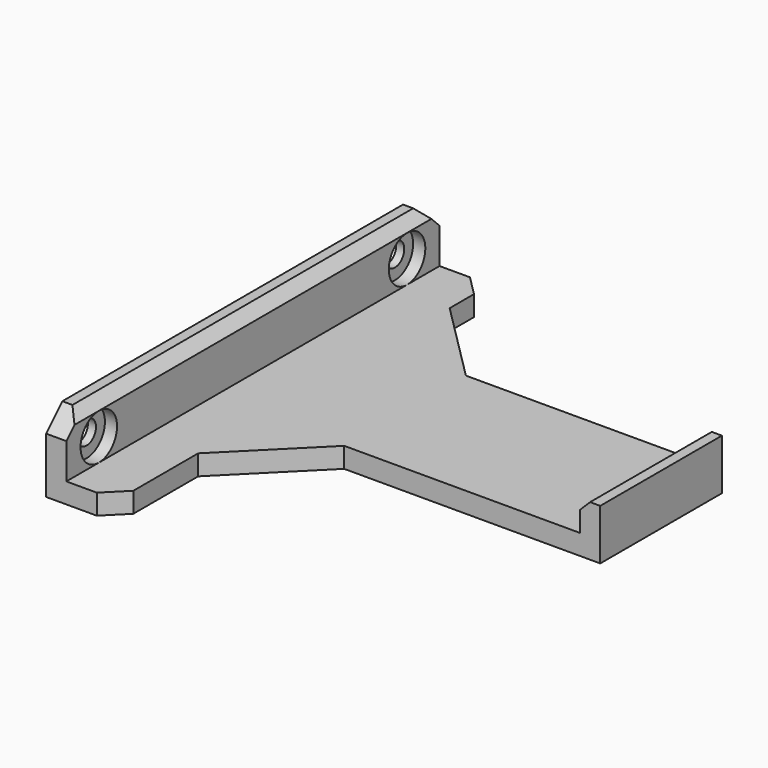
from build123d import *

# Parameters (mm, degrees)
F2_DEPTH  = 4
F3_W      = 4
F3_H      = 30
F4_DEPTH  = 6
F5_SIZE   = 16
F6_SIZE   = 2
F7_SIZE   = 4
F8_W      = 4
F8_H      = 92
F9_DEPTH  = 11
F10_R     = 4.5
F11_DEPTH = 2.4
F12_R     = 2.3
F13_DEPTH = 4
F14_SIZE  = 4
F15_SIZE  = 1.99999


# Not quite as in the source:
# - a fillet or chamfer is up to 0.001 mm smaller than in the source, because OpenCascade refuses the exact size


with BuildPart() as f2:
    # F1 (on Top) → F2 (new body)
    with BuildSketch(Plane.XY):
        Polygon((10, 46), (-4, 46), (-4, -46), (10, -46), (10, -10), (76.5, -10), (76.5, 20), (10, 20), align=None)
    extrude(amount=F2_DEPTH)

    # F3 (on face) → F4 (join)
    with BuildSketch(Plane.XY.offset(4)):
        with Locations((74.5, 5)):
            Rectangle(F3_W, F3_H)
    extrude(amount=F4_DEPTH)

    # F5
    f5_edges = [f2.edges().sort_by_distance(p)[0] for p in [
        (10, 20, 2),
        (10, -10, 2),
    ]]
    chamfer(f5_edges, length=F5_SIZE)

    # F6
    f6_edges = [f2.edges().sort_by_distance(p)[0] for p in [
        (72.5, 5, 10),
    ]]
    chamfer(f6_edges, length=F6_SIZE)

    # F7
    f7_edges = [f2.edges().sort_by_distance(p)[0] for p in [
        (10, -46, 2),
        (10, 46, 2),
    ]]
    chamfer(f7_edges, length=F7_SIZE)

    # F8 (on face) → F9 (join)
    with BuildSketch(Plane.XY.offset(4)):
        with Locations((-2, 0)):
            Rectangle(F8_W, F8_H)
    extrude(amount=F9_DEPTH)

    # F10 (on face) → F11 (cut)
    with BuildSketch(Plane.YZ):
        with Locations((-38, 8.5)):
            Circle(F10_R)
        with Locations((38, 8.5)):
            Circle(F10_R)
    extrude(amount=-F11_DEPTH, mode=Mode.SUBTRACT)

    # F12 (on face) → F13 (cut, through all)
    with BuildSketch(Plane(origin=(-4, 0, 0), x_dir=(0, -1, 0), z_dir=(-1, 0, 0))):
        with Locations((-38, 8.5)):
            Circle(F12_R)
        with Locations((38, 8.5)):
            Circle(F12_R)
    extrude(amount=-F13_DEPTH, mode=Mode.SUBTRACT)

    # F14
    f14_edges = [f2.edges().sort_by_distance(p)[0] for p in [
        (-2, -46, 15),
        (-2, 46, 15),
    ]]
    chamfer(f14_edges, length=F14_SIZE)

    # F15 (size 2 in the source; OpenCascade refuses exactly that, so slightly less here)
    f15_edges = [f2.edges().sort_by_distance(p)[0] for p in [
        (0, 0, 15),
    ]]
    chamfer(f15_edges, length=F15_SIZE)


solid = f2.part
